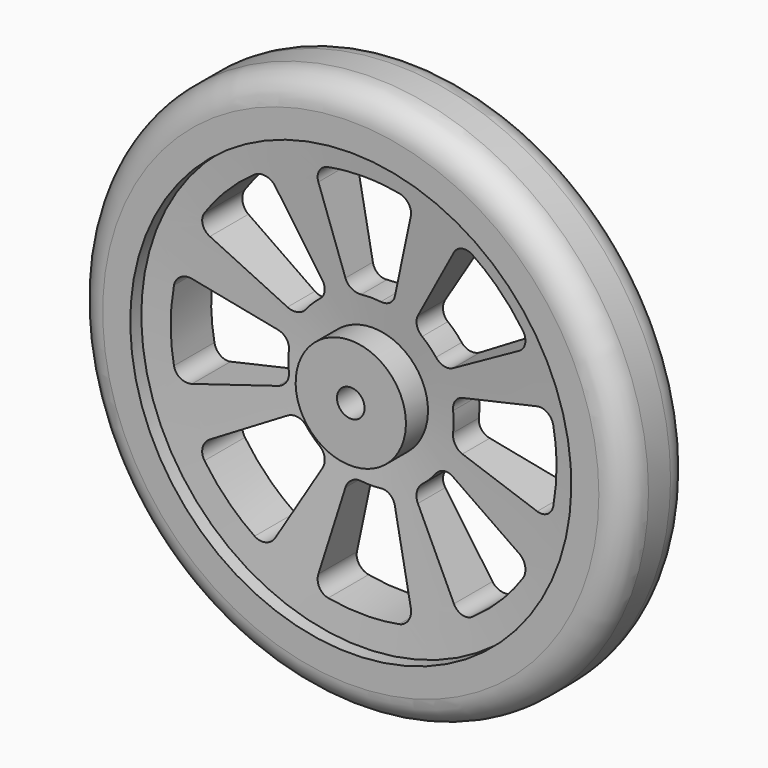
from build123d import *

# Parameters (mm, degrees)
F0_R            = 100
F1_DEPTH        = 15
F1_DEPTH_BACK   = 15
F2_R            = 10
F7_DEPTH        = 15.001
F7_DEPTH_BACK   = 15.001
F7_COPIES_COUNT = 8
F8_R            = 5
F9_DEPTH        = 30.001


# Not quite as in the source:
# - a pattern or mirror of a feature is missing from the dataset's text; its kind, count and spacing are read off the source's solid


with BuildPart() as f1:
    # F0 (on Front) → F1 (new body, two sides)
    with BuildSketch(Plane.XZ) as f1_sk:
        Circle(F0_R)
    extrude(amount=F1_DEPTH)
    extrude(f1_sk.sketch, amount=-F1_DEPTH_BACK)

    # F2
    f2_edges = [f1.edges().sort_by_distance(p)[0] for p in [
        (-100, -15, 0),
        (-100, 15, 0),
    ]]
    fillet(f2_edges, radius=F2_R)

    # F3 (on Right) → F5 (revolve, cut)
    with BuildSketch(Plane.YZ):
        Polygon((-5, 20), (-10, 80), (-15, 80), (-15, 20), align=None)
    f5 = revolve(axis=Axis((0, 0, 0), (0, -1, 0)), mode=Mode.SUBTRACT)

    # F5_copies: F5 across plane
    add(f5.mirror(Plane.ZX), mode=Mode.SUBTRACT)

    # F6 (on Front) → F7 (cut, two sides)
    with BuildSketch(Plane.XZ) as f7_sk:
        with BuildLine():
            ThreePointArc((-3.5452505059, 29.7897834643), (0, 30), (3.5452505059, 29.7897834643))
            ThreePointArc((3.5452505059, 29.7897834643), (6.9397978596, 30.6147688961), (8.9657547217, 33.4606521495))
            Line((8.9657547217, 33.4606521495), (16.7733911912, 62.5991481407))
            ThreePointArc((16.7733911912, 62.5991481407), (16.1744552307, 66.5580576738), (12.8625129874, 68.8081082406))
            ThreePointArc((12.8625129874, 68.8081082406), (0, 70), (-12.8625129874, 68.8081082406))
            ThreePointArc((-12.8625129874, 68.8081082406), (-16.1744552307, 66.5580576738), (-16.7733911912, 62.5991481407))
            Line((-16.7733911912, 62.5991481407), (-8.9657547217, 33.4606521495))
            ThreePointArc((-8.9657547217, 33.4606521495), (-6.9397978596, 30.6147688961), (-3.5452505059, 29.7897834643))
        make_face()
    f7 = extrude(amount=-F7_DEPTH, mode=Mode.SUBTRACT) + extrude(f7_sk.sketch, amount=F7_DEPTH_BACK, mode=Mode.SUBTRACT)

    # F7_copies: F7 ×8 about axis
    f7_copies_axis = Axis((0, 0, 0), (0, 1, 0))
    for i in range(1, F7_COPIES_COUNT):
        add(f7.rotate(f7_copies_axis, i * 360 / F7_COPIES_COUNT), mode=Mode.SUBTRACT)

    # F8 (on face) → F9 (cut, through all)
    with BuildSketch(Plane.XZ.offset(15)):
        Circle(F8_R)
    extrude(amount=-F9_DEPTH, mode=Mode.SUBTRACT)


solid = f1.part
